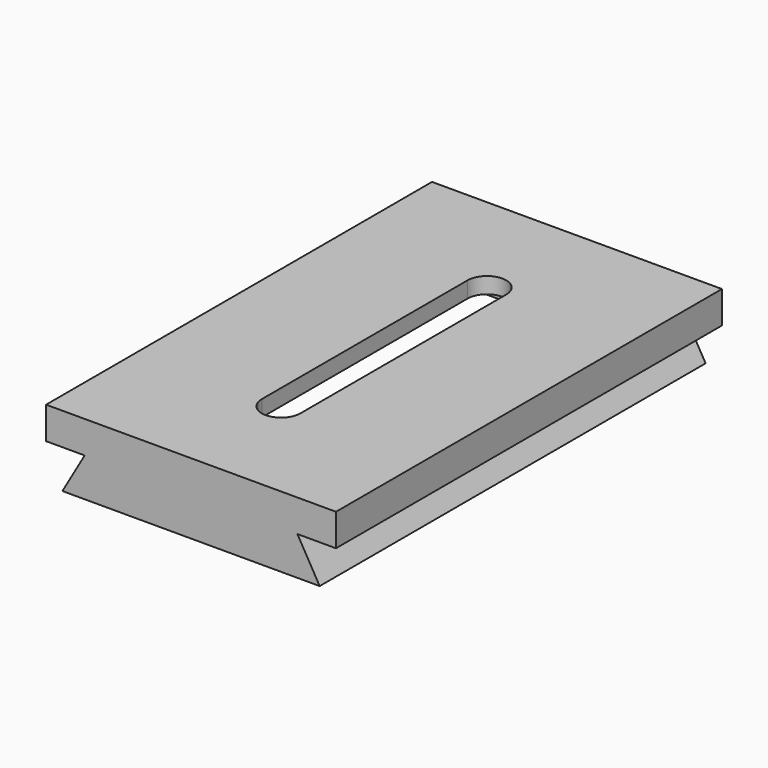
from build123d import *

# Parameters (mm, degrees)
F1_DEPTH    = 37.5
F2_T        = 2.5
F2_T3_DEPTH = 80
F4_DEPTH    = 2.5


# Not quite as in the source:
# - a shell that OpenCascade refuses in one call is made with other operations: the cavity is built on its own and cut out


with BuildPart() as f1:
    # F0 (on Front) → F1 (new body, symmetric)
    with BuildSketch(Plane.XZ):
        Polygon((-20, -3), (20, -3), (16.5358983849, 3), (22.5358983849, 3), (22.5358983849, 8), (-22.5358983849, 8), (-22.5358983849, 3), (-16.5358983849, 3), align=None)
    extrude(amount=F1_DEPTH, both=True)

    # F2: shell of thickness 2.5, made by hand


with BuildPart() as f2_core1:
    # F2_t2: copy of F1
    add(f1.part)

    # the walls: a layer under each face that stays
    f2_faces = [f2_core1.faces().sort_by_distance(p)[0] for p in [
        (-18.2679491924, 0, 0),
        (-19.5358983849, 0, 3),
        (-22.5358983849, 0, 5.5),
        (0, 0, 8),
        (22.5358983849, 0, 5.5),
        (19.5358983849, 0, 3),
        (18.2679491924, 0, 0),
        (0, -37.5, 2.5),
        (0, 37.5, 2.5),
    ]]
    thicken(f2_faces, amount=-F2_T, mode=Mode.SUBTRACT)

    # F2_s4 → F2_t3 (cut)
    with BuildSketch(Plane.XZ.offset(-40)):
        Polygon((-16.55754902, 2.9875), (-14.3708348754, 1.75), (-12.2057713659, 5.5), (-16.5358983849, 5.5), align=None)
        Polygon((16.55754902, 2.9875), (16.5358983849, 5.5), (12.2057713659, 5.5), (14.3708348754, 1.75), align=None)
    extrude(amount=F2_T3_DEPTH, mode=Mode.SUBTRACT)


with BuildPart() as f1_1:
    add(f1.part)

    # what is left inside the walls is the cavity
    f2_cavity = [f2_core1.part.solids().sort_by_distance(p)[0] for p in [
        (0, 11.666667, -2.975),
    ]]
    add(f2_cavity, mode=Mode.SUBTRACT)

    # F3 (on face) → F4 (cut, through all)
    with BuildSketch(Plane(origin=(0, 0, 5.5), x_dir=(1, 0, 0), z_dir=(0, 0, -1))):
        with BuildLine():
            Line((3, -20), (3, 20))
            ThreePointArc((3, 20), (0, 23), (-3, 20))
            Line((-3, 20), (-3, -20))
            ThreePointArc((-3, -20), (0, -23), (3, -20))
        make_face()
    extrude(amount=-F4_DEPTH, mode=Mode.SUBTRACT)


solid = f1_1.part
